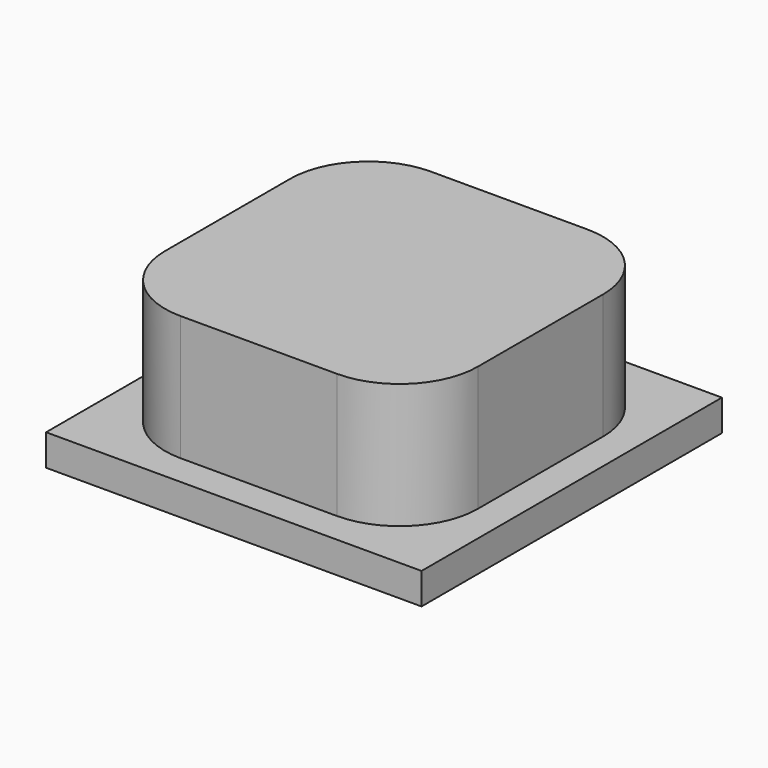
from build123d import *

# Parameters (mm, degrees)
F0_W     = 20
F0_H     = 20
F0_W_2   = 4
F0_H_2   = 4
F0_R     = 1.6
F1_DEPTH = 10
F0_W_3   = 24
F0_H_3   = 24
F2_DEPTH = 2
F3_DEPTH = 5
F5_R     = 5
F6_R     = 5
F7_R     = 1


# Not quite as in the source:
# - the program builds the solid bodies; features that only make, move or delete a surface that nothing else refers to are left out


with BuildPart() as f1:
    # F0 (on Top) → F1 (new body)
    with BuildSketch(Plane.XY):
        Rectangle(F0_W, F0_H)
        Rectangle(F0_W_2, F0_H_2, mode=Mode.SUBTRACT)
        Rectangle(F0_W_2, F0_H_2)
        Circle(F0_R, mode=Mode.SUBTRACT)
        Circle(F0_R)
    extrude(amount=F1_DEPTH)

    # F0 (on Top) → F2 (join)
    with BuildSketch(Plane.XY):
        Rectangle(F0_W_3, F0_H_3)
        Rectangle(F0_W, F0_H, mode=Mode.SUBTRACT)
    extrude(amount=F2_DEPTH)

    # F0 (on Top) → F3 (join)
    with BuildSketch(Plane.XY):
        Rectangle(F0_W_2, F0_H_2)
        Circle(F0_R, mode=Mode.SUBTRACT)
        Circle(F0_R)
    extrude(amount=-F3_DEPTH)

    # F5
    f5_edges = [f1.edges().sort_by_distance(p)[0] for p in [
        (-10, -10, 6),
    ]]
    fillet(f5_edges, radius=F5_R)

    # F6
    f6_edges = [f1.edges().sort_by_distance(p)[0] for p in [
        (10, -10, 6),
        (10, 10, 6),
        (-10, 10, 6),
    ]]
    fillet(f6_edges, radius=F6_R)

    # F7
    f7_edges = [f1.edges().sort_by_distance(p)[0] for p in [
        (2, 2, -2.5),
        (2, -2, -2.5),
        (-2, -2, -2.5),
        (-2, 2, -2.5),
    ]]
    fillet(f7_edges, radius=F7_R)


solid = f1.part
